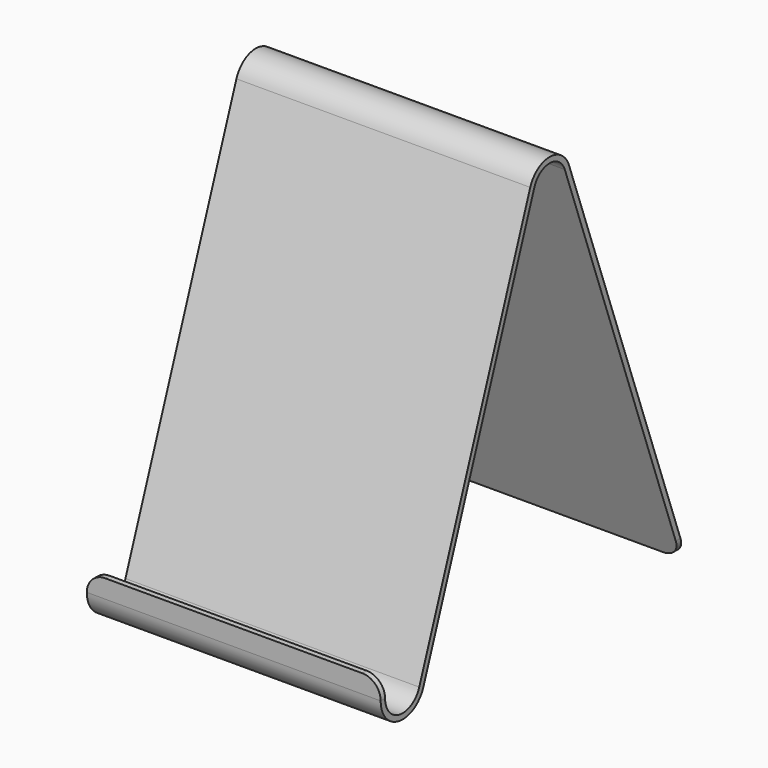
from build123d import *

# Parameters (mm, degrees)
F1_DEPTH     = 40
F2_T1_DEPTH  = 26.5951332913
F2_T6_DEPTH  = 26.5
F2_T11_DEPTH = 26.5


# Not quite as in the source:
# - a fillet or chamfer that OpenCascade refuses, or shapes differently, is made with other operations: its cross-section is extruded or revolved along the edge and cut away or added


with BuildPart() as f1:
    # F0 (on Right) → F1 (new body, symmetric)
    with BuildSketch(Plane.YZ):
        with BuildLine():
            Line((-7.5, 5), (-7.5, 0))
            ThreePointArc((-7.5, 0), (-1.2951320089, -7.3873292251), (7.0527021545, -2.5513510773))
            Line((7.0527021545, -2.5513510773), (44.82801842, 101.87099079))
            ThreePointArc((44.82801842, 101.87099079), (50, 105.5), (55.17198158, 101.87099079))
            Line((55.17198158, 101.87099079), (94.7374969044, -7.5))
            Line((94.7374969044, -7.5), (96.3326301957, -7.5))
            Line((96.3326301957, -7.5), (56.5825220109, 102.3812610054))
            ThreePointArc((56.5825220109, 102.3812610054), (50, 107), (43.4174779891, 102.3812610054))
            Line((43.4174779891, 102.3812610054), (5.6421617236, -2.0410808618))
            ThreePointArc((5.6421617236, -2.0410808618), (-1.0361056071, -5.9098633801), (-6, 0))
            Line((-6, 0), (-6, 5))
            Line((-6, 5), (-7.5, 5))
        make_face()
    extrude(amount=F1_DEPTH, both=True)

    # F2: fillet of radius 5 on 4 edges, made by hand

    # F2_s2 → F2_t1 (cut)
    with BuildSketch(Plane.XZ.offset(-108.8326301957)):
        with BuildLine():
            ThreePointArc((-35, -7.5), (-38.5355339059, -6.0355339059), (-40, -2.5))
            Line((-40, -2.5), (-40, -7.5))
            Line((-40, -7.5), (-35, -7.5))
        make_face()
        with BuildLine():
            ThreePointArc((35, -7.5), (38.5355339059, -6.0355339059), (40, -2.5))
            Line((40, -2.5), (40, -7.5))
            Line((40, -7.5), (35, -7.5))
        make_face()
    extrude(amount=F2_T1_DEPTH, mode=Mode.SUBTRACT)


with BuildPart() as f2_tool4:
    # F2_s5 → F2_t6 (new body)
    with BuildSketch(Plane.XZ.offset(-6.5)):
        with BuildLine():
            ThreePointArc((35, 5), (38.5355339059, 3.5355339059), (40, 0))
            Line((40, 0), (40, 5))
            Line((40, 5), (35, 5))
        make_face()
    extrude(amount=F2_T6_DEPTH)

    split(bisect_by=Plane(origin=(0, 5.6421617236, -2.0410808618), x_dir=(1, 0, 0), z_dir=(0, -0.9403602873, 0.3401801436)), keep=Keep.TOP)


with BuildPart() as f1_1:
    add(f1.part)

    # F2_t3: cut F2_tool4
    add(f2_tool4.part, mode=Mode.SUBTRACT)


with BuildPart() as f2_tool9:
    # F2_s10 → F2_t11 (new body)
    with BuildSketch(Plane.XZ.offset(-6.5)):
        with BuildLine():
            ThreePointArc((-35, 5), (-38.5355339059, 3.5355339059), (-40, 0))
            Line((-40, 0), (-40, 5))
            Line((-40, 5), (-35, 5))
        make_face()
    extrude(amount=F2_T11_DEPTH)

    split(bisect_by=Plane(origin=(0, 5.6421617236, -2.0410808618), x_dir=(1, 0, 0), z_dir=(0, -0.9403602873, 0.3401801436)), keep=Keep.TOP)


with BuildPart() as f1_2:
    add(f1_1.part)

    # F2_t8: cut F2_tool9
    add(f2_tool9.part, mode=Mode.SUBTRACT)


solid = f1_2.part
